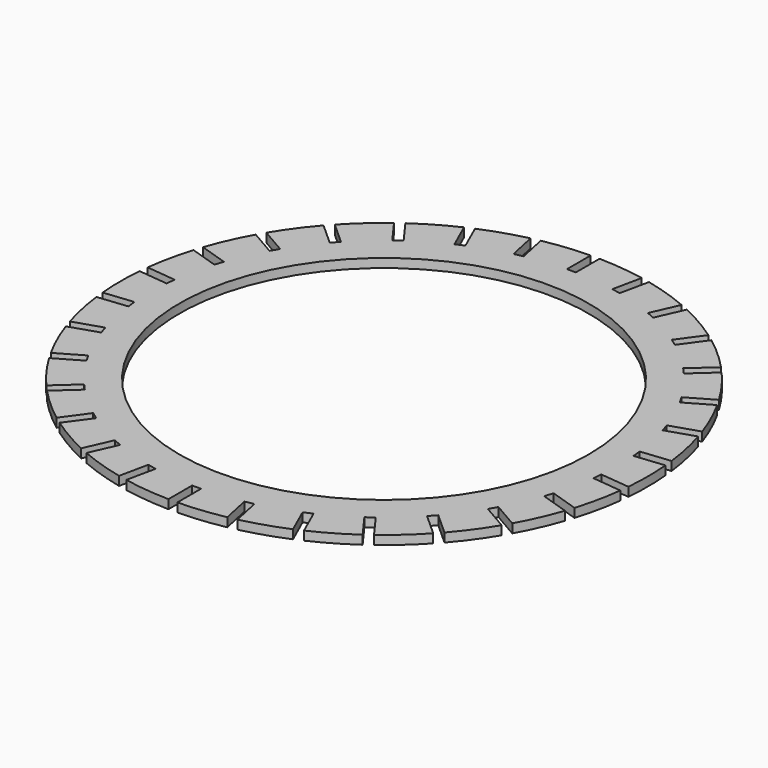
from build123d import *

# Parameters (mm, degrees)
F0_R            = 89
F0_R_2          = 69
F1_DEPTH        = 3
F3_DEPTH        = 25
F3_COPIES_COUNT = 30


# Not quite as in the source:
# - a pattern or mirror of a feature is missing from the dataset's text; its kind, count and spacing are read off the source's solid


with BuildPart() as f1:
    # F0 (on Top) → F1 (new body)
    with BuildSketch(Plane.XY):
        Circle(F0_R)
        Circle(F0_R_2, mode=Mode.SUBTRACT)
    extrude(amount=F1_DEPTH)

    # F2 (on Top) → F3 (cut)
    with BuildSketch(Plane.XY):
        Polygon((-1.5, -89), (0, -89), (1.5, -89), (1.5, -79), (-1.5, -79), align=None)
    f3 = extrude(amount=F3_DEPTH, mode=Mode.SUBTRACT)

    # F3_copies: F3 ×30 about axis
    f3_copies_axis = Axis((0, 0, 0), (0, 0, 1))
    for i in range(1, F3_COPIES_COUNT):
        add(f3.rotate(f3_copies_axis, i * 360 / F3_COPIES_COUNT), mode=Mode.SUBTRACT)


solid = f1.part
